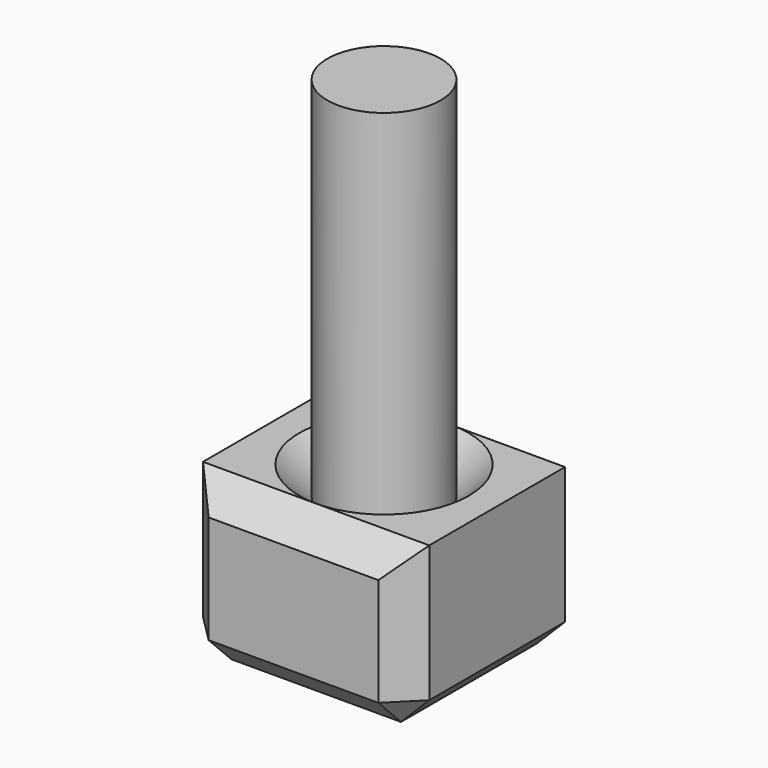
from build123d import *

# Parameters (mm, degrees)
F0_W     = 40
F0_H     = 40
F0_R     = 10
F1_DEPTH = 29.1
F2_DEPTH = 89
F3_SIZE  = 4.99999


# Not quite as in the source:
# - a fillet or chamfer is up to 0.001 mm smaller than in the source, because OpenCascade refuses the exact size


with BuildPart() as f1:
    # F0 (on Top) → F1 (new body)
    with BuildSketch(Plane.XY):
        Rectangle(F0_W, F0_H)
        Circle(F0_R, mode=Mode.SUBTRACT)
    extrude(amount=F1_DEPTH)

    # F3 (size 5 in the source; OpenCascade refuses exactly that, so slightly less here)
    f3_edges = [f1.edges().sort_by_distance(p)[0] for p in [
        (0, -20, 29.1),
        (0, -20, 0),
        (-20, -20, 14.55),
        (20, -20, 14.55),
        (20, 20, 14.55),
        (-20, 20, 14.55),
        (0, 20, 0),
        (0, 20, 29.1),
        (-10, 0, 29.1),
        (20, 0, 0),
        (-20, 0, 0),
        (-10, 0, 0),
    ]]
    chamfer(f3_edges, length=F3_SIZE)


with BuildPart() as f2:
    # F0 (on Top) → F2 (new body)
    with BuildSketch(Plane.XY):
        Circle(F0_R)
    extrude(amount=F2_DEPTH)


solid = Compound([f1.part, f2.part])
